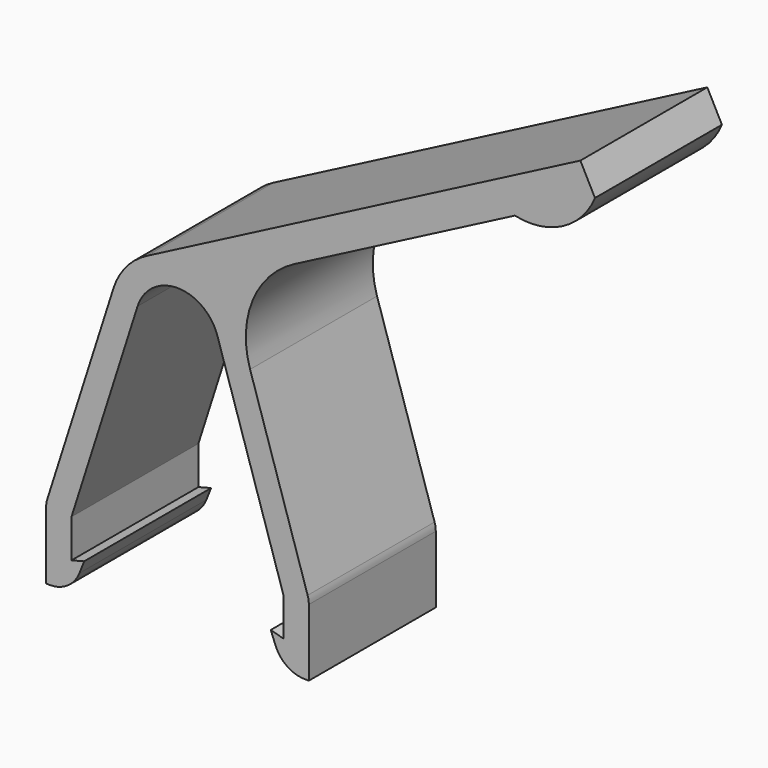
from build123d import *

# Parameters (mm, degrees)
F1_DEPTH = 12.5
F2_R     = 5


# Not quite as in the source:
# - a feature names something its author has since deleted; it is built from what else it names


with BuildPart() as f1:
    # F0 (on Front) → F1 (new body, symmetric)
    with BuildSketch(Plane.XZ):
        with BuildLine():
            ThreePointArc((-6.2894771713, 32.5883566917), (0, 37.1817581393), (6.2894771713, 32.5883566917))
            Line((6.2894771713, 32.5883566917), (16.7, 0))
            Line((16.7, 0), (20.7, 0))
            ThreePointArc((20.7, 0), (20.6522901201, 0.6159568218), (20.5102985969, 1.2172200305))
            Line((20.5102985969, 1.2172200305), (11.4429113124, 29.6011211997))
            ThreePointArc((11.4429113124, 29.6011211997), (11.8429318518, 39.3121369153), (18.4103098825, 46.4768691826))
            Line((18.4103098825, 46.4768691826), (53.1603869456, 64.5016425675))
            Line((53.1603869456, 64.5016425675), (65.7802901999, 71.0475531243))
            Line((65.7802901999, 71.0475531243), (63.4780788017, 75.4860013529))
            Line((63.4780788017, 75.4860013529), (-4.8740239191, 40.0319458213))
            ThreePointArc((-4.8740239191, 40.0319458213), (-8.0911004209, 37.4607846039), (-10.0835041229, 33.8565123177))
            Line((-10.0835041229, 33.8565123177), (-20.5102985969, 1.2172200305))
            ThreePointArc((-20.5102985969, 1.2172200305), (-20.6522901201, 0.6159568218), (-20.7, 0))
            Line((-20.7, 0), (-16.7, 0))
            Line((-16.7, 0), (-6.2894771713, 32.5883566917))
        make_face()
        Polygon((-16.7, -5.2822484933), (-16.7, 0), (-20.7, 0), (-20.7, -10.5644969866), (-16.7, -10.5644969866), (-16.7, -6.0322484933), align=None)
        Polygon((20.7, 0), (16.7, 0), (16.7, -5.2822484933), (16.7, -6.0322484933), (16.7, -10.5644969866), (20.7, -10.5644969866), align=None)
        with BuildLine():
            Line((65.7802901999, 71.0475531243), (53.1603869456, 64.5016425675))
            ThreePointArc((53.1603869456, 64.5016425675), (60.6653765198, 65.4706764668), (65.7802901999, 71.0475531243))
        make_face()
        Polygon((-14.7, -5.5168885775), (-16.7, -6.0322484933), (-16.7, -10.5644969866), align=None)
        Polygon((16.7, -10.5644969866), (16.7, -6.0322484933), (14.7, -5.4739810377), align=None)
    extrude(amount=F1_DEPTH, both=True)

    # F2
    f2_edges = [f1.edges().sort_by_distance(p)[0] for p in [
        (16.7, 0, -10.564497),
        (-16.7, 0, -10.564497),
    ]]
    fillet(f2_edges, radius=F2_R)


solid = f1.part
